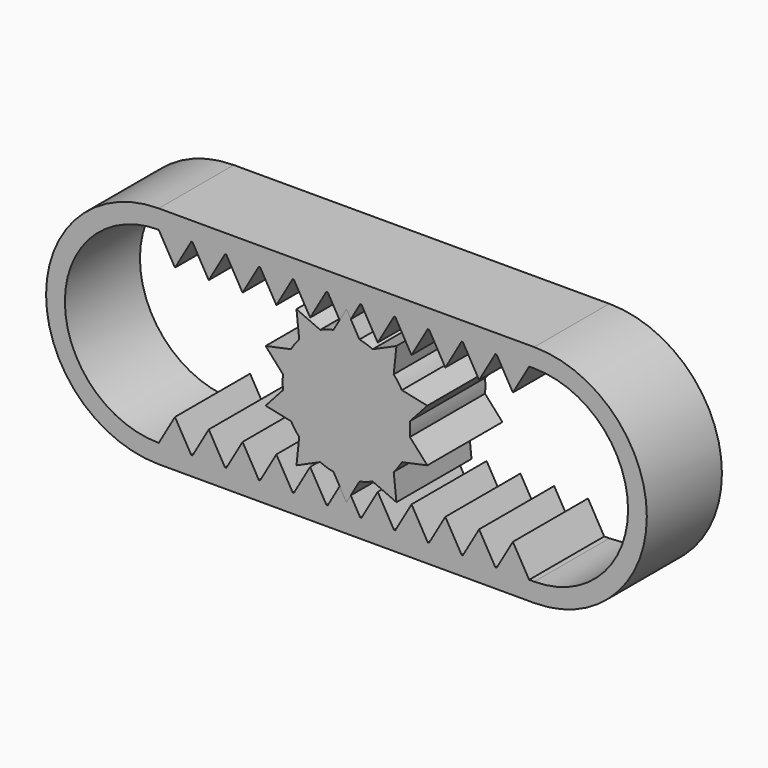
from build123d import *

# Parameters (mm, degrees)
F1_DEPTH = 12.5
F3_DEPTH = 12.5


with BuildPart() as f1:
    # F0 (on Front) → F1 (new body, symmetric)
    with BuildSketch(Plane.XZ):
        with BuildLine():
            ThreePointArc((50, -30), (80, 0), (50, 30))
            Line((50, 30), (-50, 30))
            ThreePointArc((-50, 30), (-80, 0), (-50, -30))
            Line((-50, -30), (50, -30))
        make_face()
        with BuildLine():
            Line((48.6602540378, 25), (50, 25))
            ThreePointArc((50, 25), (75, 0), (50, -25))
            Line((50, -25), (48.6602540378, -25))
            Line((48.6602540378, -25), (40, -25))
            Line((40, -25), (39.6602540378, -25))
            Line((39.6602540378, -25), (31, -25))
            Line((31, -25), (30.6602540378, -25))
            Line((30.6602540378, -25), (22, -25))
            Line((22, -25), (21.6602540378, -25))
            Line((21.6602540378, -25), (13, -25))
            Line((13, -25), (12.6602540378, -25))
            Line((12.6602540378, -25), (4, -25))
            Line((4, -25), (3.6602540378, -25))
            Line((3.6602540378, -25), (-5, -25))
            Line((-5, -25), (-5.3397459622, -25))
            Line((-5.3397459622, -25), (-14, -25))
            Line((-14, -25), (-14.3397459622, -25))
            Line((-14.3397459622, -25), (-23, -25))
            Line((-23, -25), (-23.3397459622, -25))
            Line((-23.3397459622, -25), (-32, -25))
            Line((-32, -25), (-32.3397459622, -25))
            Line((-32.3397459622, -25), (-41, -25))
            Line((-41, -25), (-41.3397459622, -25))
            Line((-41.3397459622, -25), (-50, -25))
            ThreePointArc((-50, -25), (-75, 0), (-50, 25))
            Line((-50, 25), (-41.3397459622, 25))
            Line((-41.3397459622, 25), (-41, 25))
            Line((-41, 25), (-32.3397459622, 25))
            Line((-32.3397459622, 25), (-32, 25))
            Line((-32, 25), (-23.3397459622, 25))
            Line((-23.3397459622, 25), (-23, 25))
            Line((-23, 25), (-14.3397459622, 25))
            Line((-14.3397459622, 25), (-14, 25))
            Line((-14, 25), (-5.3397459622, 25))
            Line((-5.3397459622, 25), (-5, 25))
            Line((-5, 25), (3.6602540378, 25))
            Line((3.6602540378, 25), (4, 25))
            Line((4, 25), (12.6602540378, 25))
            Line((12.6602540378, 25), (13, 25))
            Line((13, 25), (21.6602540378, 25))
            Line((21.6602540378, 25), (22, 25))
            Line((22, 25), (30.6602540378, 25))
            Line((30.6602540378, 25), (31, 25))
            Line((31, 25), (39.6602540378, 25))
            Line((39.6602540378, 25), (40, 25))
            Line((40, 25), (48.6602540378, 25))
        make_face(mode=Mode.SUBTRACT)
        Polygon((44.3301270189, 17.5), (48.6602540378, 25), (40, 25), align=None)
        Polygon((40, -25), (48.6602540378, -25), (44.3301270189, -17.5), align=None)
        Polygon((35.3301270189, 17.5), (39.6602540378, 25), (31, 25), align=None)
        Polygon((31, -25), (39.6602540378, -25), (35.3301270189, -17.5), align=None)
        Polygon((26.3301270189, 17.5), (30.6602540378, 25), (22, 25), align=None)
        Polygon((22, -25), (30.6602540378, -25), (26.3301270189, -17.5), align=None)
        Polygon((17.3301270189, 17.5), (21.6602540378, 25), (13, 25), align=None)
        Polygon((13, -25), (21.6602540378, -25), (17.3301270189, -17.5), align=None)
        Polygon((8.3301270189, 17.5), (12.6602540378, 25), (4, 25), align=None)
        Polygon((4, -25), (12.6602540378, -25), (8.3301270189, -17.5), align=None)
        Polygon((-0.6698729811, 17.5), (3.6602540378, 25), (-5, 25), align=None)
        Polygon((-5, -25), (3.6602540378, -25), (-0.6698729811, -17.5), align=None)
        Polygon((-9.6698729811, 17.5), (-5.3397459622, 25), (-14, 25), align=None)
        Polygon((-14, -25), (-5.3397459622, -25), (-9.6698729811, -17.5), align=None)
        Polygon((-18.6698729811, 17.5), (-14.3397459622, 25), (-23, 25), align=None)
        Polygon((-23, -25), (-14.3397459622, -25), (-18.6698729811, -17.5), align=None)
        Polygon((-27.6698729811, 17.5), (-23.3397459622, 25), (-32, 25), align=None)
        Polygon((-32, -25), (-23.3397459622, -25), (-27.6698729811, -17.5), align=None)
        Polygon((-36.6698729811, 17.5), (-32.3397459622, 25), (-41, 25), align=None)
        Polygon((-41, -25), (-32.3397459622, -25), (-36.6698729811, -17.5), align=None)
        Polygon((-45.6698729811, 17.5), (-41.3397459622, 25), (-50, 25), align=None)
        Polygon((-50, -25), (-41.3397459622, -25), (-45.6698729811, -17.5), align=None)
    extrude(amount=F1_DEPTH, both=True)


with BuildPart() as f3:
    # F2 (on Front) → F3 (new body, symmetric)
    with BuildSketch(Plane.XZ):
        with BuildLine():
            Line((0, 22.6433169771), (-3.4641016151, 16.6433169771))
            ThreePointArc((-3.4641016151, 16.6433169771), (-5.2532889044, 16.167960777), (-6.9801791915, 15.5008741191))
            ThreePointArc((-6.9801791915, 15.5008741191), (-9.992349289, 13.7532889044), (-12.5852133453, 11.4285784354))
            ThreePointArc((-12.5852133453, 11.4285784354), (-13.7532889044, 9.992349289), (-14.7582687945, 8.4376242029))
            Line((-14.7582687945, 8.4376242029), (-21.5350741616, 6.9971697549))
            Line((-21.5350741616, 6.9971697549), (-16.8992013331, 1.8485113745))
            ThreePointArc((-16.8992013331, 1.8485113745), (-17, 0), (-16.8992013331, -1.8485113745))
            Line((-16.8992013331, -1.8485113745), (-21.5350741616, -6.9971697549))
            Line((-21.5350741616, -6.9971697549), (-14.7582687945, -8.4376242029))
            ThreePointArc((-14.7582687945, -8.4376242029), (-13.7532889044, -9.992349289), (-12.5852133453, -11.4285784354))
            Line((-12.5852133453, -11.4285784354), (-13.3094077821, -18.3188282435))
            Line((-13.3094077821, -18.3188282435), (-6.9801791915, -15.5008741191))
            ThreePointArc((-6.9801791915, -15.5008741191), (-5.2532889044, -16.167960777), (-3.4641016151, -16.6433169771))
            Line((-3.4641016151, -16.6433169771), (0, -22.6433169771))
            Line((0, -22.6433169771), (3.4641016151, -16.6433169771))
            ThreePointArc((3.4641016151, -16.6433169771), (5.2532889044, -16.167960777), (6.9801791915, -15.5008741191))
            Line((6.9801791915, -15.5008741191), (13.3094077821, -18.3188282435))
            Line((13.3094077821, -18.3188282435), (12.5852133453, -11.4285784354))
            ThreePointArc((12.5852133453, -11.4285784354), (13.7532889044, -9.992349289), (14.7582687945, -8.4376242029))
            Line((14.7582687945, -8.4376242029), (21.5350741616, -6.9971697549))
            Line((21.5350741616, -6.9971697549), (16.8992013331, -1.8485113745))
            ThreePointArc((16.8992013331, -1.8485113745), (17, 0), (16.8992013331, 1.8485113745))
            Line((16.8992013331, 1.8485113745), (21.5350741616, 6.9971697549))
            Line((21.5350741616, 6.9971697549), (14.7582687945, 8.4376242029))
            ThreePointArc((14.7582687945, 8.4376242029), (13.7532889044, 9.992349289), (12.5852133453, 11.4285784354))
            Line((12.5852133453, 11.4285784354), (13.3094077821, 18.3188282435))
            Line((13.3094077821, 18.3188282435), (6.9801791915, 15.5008741191))
            ThreePointArc((6.9801791915, 15.5008741191), (5.2532889044, 16.167960777), (3.4641016151, 16.6433169771))
            Line((3.4641016151, 16.6433169771), (0, 22.6433169771))
        make_face()
        with BuildLine():
            ThreePointArc((-12.5852133453, 11.4285784354), (-9.992349289, 13.7532889044), (-6.9801791915, 15.5008741191))
            Line((-6.9801791915, 15.5008741191), (-13.3094077821, 18.3188282435))
            Line((-13.3094077821, 18.3188282435), (-12.5852133453, 11.4285784354))
        make_face()
    extrude(amount=F3_DEPTH, both=True)


solid = Compound([f1.part, f3.part])
